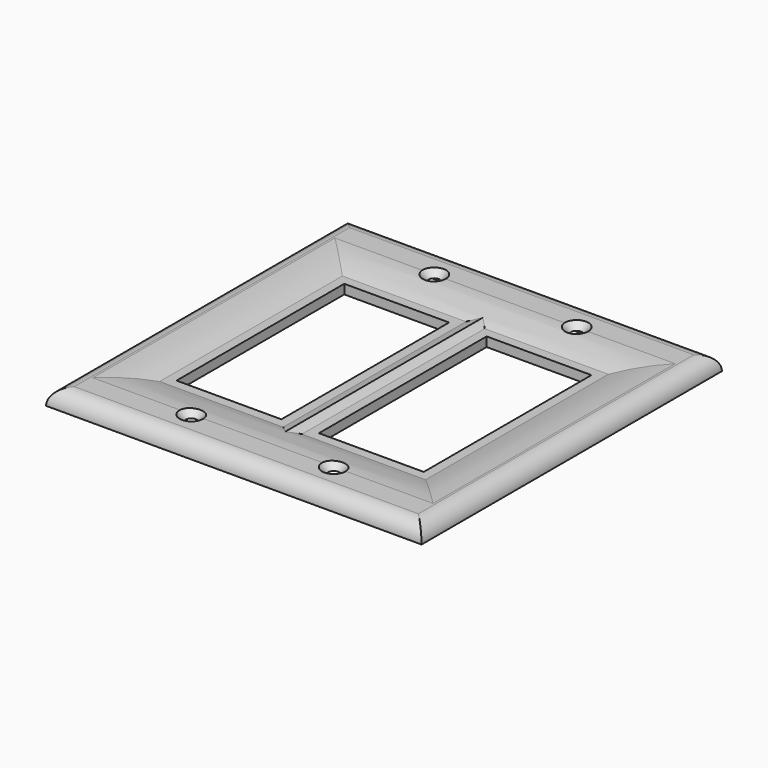
from build123d import *

# Parameters (mm, degrees)
F0_R          = 1.75
F0_W          = 39.5000008941
F0_H          = 73.0000008941
F0_W_2        = 33.5
F0_H_2        = 67
F1_DEPTH      = 5
F2_DEPTH      = 3
F3_R          = 4.99999
F4_R          = 1.5
F5_SIZE       = 1.99999
F6_R          = 2.99999
F7_START      = 3
F7_DEPTH      = 22
F8_T1_DEPTH   = 73.0000008941
F8_T3_DEPTH   = 39.5000008941
F8_T5_DEPTH   = 39.5000008941
F8_T10_DEPTH  = 69.1703579174
F8_T15_DEPTH  = 69.1703579174
F8_T20_DEPTH  = 69.1703579174
F8_T25_DEPTH  = 69.1703579174
F8_T31_DEPTH  = 102.6703579174
F8_T35_DEPTH  = 69.1703579174
F8_T43_DEPTH  = 69.1703579174
F8_T48_DEPTH  = 102.6703579174
F8_T55_DEPTH  = 102.6703579174
F8_T59_DEPTH  = 69.1703579174
F8_T66_DEPTH  = 69.1703579174
F8_T71_DEPTH  = 102.6703579174
F8_T78_DEPTH  = 102.6703579174
F8_T82_DEPTH  = 69.1703579174
F8_T89_DEPTH  = 69.1703579174
F8_T93_DEPTH  = 102.6703579174
F8_T100_DEPTH = 69.1703579174
F8_T105_DEPTH = 102.6703579174
F8_T112_DEPTH = 102.6703579174
F8_T116_DEPTH = 69.1703579174


# Not quite as in the source:
# - a fillet or chamfer that OpenCascade refuses, or shapes differently, is made with other operations: its cross-section is extruded or revolved along the edge and cut away or added
# - a fillet or chamfer is up to 0.001 mm smaller than in the source, because OpenCascade refuses the exact size
# - a feature names something its author has since deleted; it is built from what else it names


with BuildPart() as f1:
    # F0 (on Top) → F1 (new body)
    with BuildSketch(Plane.XY):
        Polygon((-60, -60), (60, -60), (60, 60), (-6, 60), (-60, 60), align=None)
        Polygon((-54.0000014007, 54.0000014007), (-6, 54.0000014007), (54.0000014007, 54.0000014007), (54.0000014007, -54.0000014007), (-54.0000014007, -54.0000014007), align=None, mode=Mode.SUBTRACT)
        Polygon((54.0000014007, 54.0000014007), (-6, 54.0000014007), (-54.0000014007, 54.0000014007), (-54.0000014007, -54.0000014007), (54.0000014007, -54.0000014007), align=None)
        with Locations((-22.75, -48.5)):
            Circle(F0_R, mode=Mode.SUBTRACT)
        with Locations((22.75, -48.5)):
            Circle(F0_R, mode=Mode.SUBTRACT)
        Polygon((-42.500000447, 36.500000447), (-6, 36.500000447), (-2.999999553, 36.500000447), (-2.999999553, -36.500000447), (-42.500000447, -36.500000447), align=None, mode=Mode.SUBTRACT)
        with Locations((-22.75, 48.5)):
            Circle(F0_R, mode=Mode.SUBTRACT)
        with Locations((22.75, 0)):
            Rectangle(F0_W, F0_H, mode=Mode.SUBTRACT)
        with Locations((22.75, 48.5)):
            Circle(F0_R, mode=Mode.SUBTRACT)
        Polygon((-2.999999553, 36.500000447), (-6, 36.500000447), (-42.500000447, 36.500000447), (-42.500000447, -36.500000447), (-2.999999553, -36.500000447), align=None)
        with Locations((-22.75, 0)):
            Rectangle(F0_W_2, F0_H_2, mode=Mode.SUBTRACT)
        with Locations((22.75, 0)):
            Rectangle(F0_W, F0_H)
        with Locations((22.75, 0)):
            Rectangle(F0_W_2, F0_H_2, mode=Mode.SUBTRACT)
    extrude(amount=F1_DEPTH)

    # F0 (on Top) → F2 (cut)
    with BuildSketch(Plane.XY):
        Polygon((54.0000014007, 54.0000014007), (-6, 54.0000014007), (-54.0000014007, 54.0000014007), (-54.0000014007, -54.0000014007), (54.0000014007, -54.0000014007), align=None)
        with Locations((-22.75, -48.5)):
            Circle(F0_R, mode=Mode.SUBTRACT)
        with Locations((22.75, -48.5)):
            Circle(F0_R, mode=Mode.SUBTRACT)
        Polygon((-42.500000447, 36.500000447), (-6, 36.500000447), (-2.999999553, 36.500000447), (-2.999999553, -36.500000447), (-42.500000447, -36.500000447), align=None, mode=Mode.SUBTRACT)
        with Locations((-22.75, 48.5)):
            Circle(F0_R, mode=Mode.SUBTRACT)
        with Locations((22.75, 0)):
            Rectangle(F0_W, F0_H, mode=Mode.SUBTRACT)
        with Locations((22.75, 48.5)):
            Circle(F0_R, mode=Mode.SUBTRACT)
    extrude(amount=F2_DEPTH, mode=Mode.SUBTRACT)

    # F3 (radius 5 in the source; OpenCascade refuses exactly that, so slightly less here)
    f3_edges = [f1.edges().sort_by_distance(p)[0] for p in [
        (0, -60, 5),
        (60, 0, 5),
        (-60, 0, 5),
        (0, 60, 5),
    ]]
    fillet(f3_edges, radius=F3_R)

    # F4
    f4_edges = [f1.edges().sort_by_distance(p)[0] for p in [
        (0, 54.000001, 3),
        (54.000001, 0, 3),
        (0, -54.000001, 3),
        (-54.000001, 0, 3),
    ]]
    fillet(f4_edges, radius=F4_R)

    # F5 (size 2 in the source; OpenCascade refuses exactly that, so slightly less here)
    f5_edges = [f1.edges().sort_by_distance(p)[0] for p in [
        (-24.5, -48.5, 5),
        (21, -48.5, 5),
        (-24.5, 48.5, 5),
        (21, 48.5, 5),
    ]]
    chamfer(f5_edges, length=F5_SIZE)

    # F6 (radius 3 in the source; OpenCascade refuses exactly that, so slightly less here)
    f6_edges = [f1.edges().sort_by_distance(p)[0] for p in [
        (22.75, 36.5, 3),
        (42.5, 0, 3),
        (-22.75, 36.5, 3),
        (-42.5, 0, 3),
        (-22.75, -36.5, 3),
        (22.75, -36.5, 3),
        (3, 0, 3),
        (-3, 0, 3),
    ]]
    fillet(f6_edges, radius=F6_R)

    # F0 (on Top) → F7 (cut)
    with BuildSketch(Plane.XY.offset(F7_START)):
        Polygon((-2.999999553, 36.500000447), (-6, 36.500000447), (-42.500000447, 36.500000447), (-42.500000447, -36.500000447), (-2.999999553, -36.500000447), align=None)
        with Locations((-22.75, 0)):
            Rectangle(F0_W_2, F0_H_2, mode=Mode.SUBTRACT)
        with Locations((22.75, 0)):
            Rectangle(F0_W, F0_H)
        with Locations((22.75, 0)):
            Rectangle(F0_W_2, F0_H_2, mode=Mode.SUBTRACT)
    extrude(amount=F7_DEPTH, mode=Mode.SUBTRACT)

    # F8: fillet of radius 36.2132034356 on 8 edges, made by hand

    # F8_s2 → F8_t1 (cut)
    with BuildSketch(Plane.XZ.offset(-36.500000447)):
        with BuildLine():
            ThreePointArc((-8.8681432564, 5), (-2.8504025312, 4.4964997224), (2.999999553, 3))
            Line((2.999999553, 3), (2.999999553, 5))
            Line((2.999999553, 5), (-8.8681432564, 5))
        make_face()
        with BuildLine():
            ThreePointArc((-54.3681432564, 5), (-48.3504025312, 4.4964997224), (-42.500000447, 3))
            Line((-42.500000447, 3), (-42.500000447, 5))
            Line((-42.500000447, 5), (-54.3681432564, 5))
        make_face()
        with BuildLine():
            ThreePointArc((54.3681432564, 5), (48.3504025312, 4.4964997224), (42.500000447, 3))
            Line((42.500000447, 3), (42.500000447, 5))
            Line((42.500000447, 5), (54.3681432564, 5))
        make_face()
        with BuildLine():
            ThreePointArc((8.8681432564, 5), (2.8504025312, 4.4964997224), (-2.999999553, 3))
            Line((-2.999999553, 3), (-2.999999553, 5))
            Line((-2.999999553, 5), (8.8681432564, 5))
        make_face()
    extrude(amount=F8_T1_DEPTH, mode=Mode.SUBTRACT)

    # F8_s4 → F8_t3 (cut)
    with BuildSketch(Plane.YZ.offset(2.999999553)):
        with BuildLine():
            ThreePointArc((-48.3681432564, 5), (-42.3504025312, 4.4964997224), (-36.500000447, 3))
            Line((-36.500000447, 3), (-36.500000447, 5))
            Line((-36.500000447, 5), (-48.3681432564, 5))
        make_face()
        with BuildLine():
            ThreePointArc((48.3681432564, 5), (42.3504025312, 4.4964997224), (36.500000447, 3))
            Line((36.500000447, 3), (36.500000447, 5))
            Line((36.500000447, 5), (48.3681432564, 5))
        make_face()
    extrude(amount=F8_T3_DEPTH, mode=Mode.SUBTRACT)

    # F8_s6 → F8_t5 (cut)
    with BuildSketch(Plane.YZ.offset(-42.500000447)):
        with BuildLine():
            ThreePointArc((-48.3681432564, 5), (-42.3504025312, 4.4964997224), (-36.500000447, 3))
            Line((-36.500000447, 3), (-36.500000447, 5))
            Line((-36.500000447, 5), (-48.3681432564, 5))
        make_face()
        with BuildLine():
            ThreePointArc((48.3681432564, 5), (42.3504025312, 4.4964997224), (36.500000447, 3))
            Line((36.500000447, 3), (36.500000447, 5))
            Line((36.500000447, 5), (48.3681432564, 5))
        make_face()
    extrude(amount=F8_T5_DEPTH, mode=Mode.SUBTRACT)


with BuildPart() as f8_tool8:
    # F8_s9 → F8_t10 (new body)
    with BuildSketch(Plane.YZ.offset(42.500000447)):
        with BuildLine():
            ThreePointArc((-48.3681432564, 5), (-42.3504025312, 4.4964997224), (-36.500000447, 3))
            Line((-36.500000447, 3), (-36.500000447, 5))
            Line((-36.500000447, 5), (-48.3681432564, 5))
        make_face()
    extrude(amount=-F8_T10_DEPTH)

    split(bisect_by=Plane.YZ.offset(-2.999999553), keep=Keep.BOTTOM)


with BuildPart() as f1_1:
    add(f1.part)

    # F8_t7: cut F8_tool8
    add(f8_tool8.part, mode=Mode.SUBTRACT)


with BuildPart() as f8_tool13:
    # F8_s14 → F8_t15 (new body)
    with BuildSketch(Plane.YZ.offset(26.6703574704)):
        with BuildLine():
            ThreePointArc((-48.3681432564, 5), (-42.3504025312, 4.4964997224), (-36.500000447, 3))
            Line((-36.500000447, 3), (-36.500000447, 5))
            Line((-36.500000447, 5), (-48.3681432564, 5))
        make_face()
    extrude(amount=-F8_T15_DEPTH)

    split(bisect_by=Plane.YZ.offset(2.999999553), keep=Keep.TOP)


with BuildPart() as f1_2:
    add(f1_1.part)

    # F8_t12: cut F8_tool13
    add(f8_tool13.part, mode=Mode.SUBTRACT)


with BuildPart() as f8_tool18:
    # F8_s19 → F8_t20 (new body)
    with BuildSketch(Plane.YZ.offset(-42.500000447)):
        with BuildLine():
            ThreePointArc((48.3681432564, 5), (42.3504025312, 4.4964997224), (36.500000447, 3))
            Line((36.500000447, 3), (36.500000447, 5))
            Line((36.500000447, 5), (48.3681432564, 5))
        make_face()
    extrude(amount=F8_T20_DEPTH)

    split(bisect_by=Plane.YZ.offset(2.999999553), keep=Keep.TOP)


with BuildPart() as f1_3:
    add(f1_2.part)

    # F8_t17: cut F8_tool18
    add(f8_tool18.part, mode=Mode.SUBTRACT)


with BuildPart() as f8_tool23:
    # F8_s24 → F8_t25 (new body)
    with BuildSketch(Plane.YZ.offset(-26.6703574704)):
        with BuildLine():
            ThreePointArc((48.3681432564, 5), (42.3504025312, 4.4964997224), (36.500000447, 3))
            Line((36.500000447, 3), (36.500000447, 5))
            Line((36.500000447, 5), (48.3681432564, 5))
        make_face()
    extrude(amount=F8_T25_DEPTH)

    split(bisect_by=Plane.YZ.offset(-2.999999553), keep=Keep.BOTTOM)


with BuildPart() as f1_4:
    add(f1_3.part)

    # F8_t22: cut F8_tool23
    add(f8_tool23.part, mode=Mode.SUBTRACT)


with BuildPart() as f8_tool29:
    # F8_s30 → F8_t31 (new body)
    with BuildSketch(Plane.XZ.offset(66.1703574704)):
        with BuildLine():
            ThreePointArc((-8.8681432564, 5), (-2.8504025312, 4.4964997224), (2.999999553, 3))
            Line((2.999999553, 3), (2.999999553, 5))
            Line((2.999999553, 5), (-8.8681432564, 5))
        make_face()
    extrude(amount=-F8_T31_DEPTH)

    split(bisect_by=Plane.XZ.offset(36.500000447), keep=Keep.TOP)


with BuildPart() as f8_tool33:
    # F8_s34 → F8_t35 (new body)
    with BuildSketch(Plane.YZ.offset(42.500000447)):
        with BuildLine():
            ThreePointArc((-48.3681432564, 5), (-42.3504025312, 4.4964997224), (-36.500000447, 3))
            Line((-36.500000447, 3), (-36.500000447, 5))
            Line((-36.500000447, 5), (-48.3681432564, 5))
        make_face()
    extrude(amount=-F8_T35_DEPTH)

    split(bisect_by=Plane.YZ.offset(2.999999553), keep=Keep.BOTTOM)

    split(bisect_by=Plane.YZ.offset(-2.999999553), keep=Keep.TOP)


with BuildPart() as f8_tool29_1:
    add(f8_tool29.part)

    # F8_t38: intersect F8_tool33
    add(f8_tool33.part, mode=Mode.INTERSECT)


with BuildPart() as f1_5:
    add(f1_4.part)

    # F8_t27: cut F8_tool29
    add(f8_tool29_1.part, mode=Mode.SUBTRACT)


with BuildPart() as f8_tool41:
    # F8_s42 → F8_t43 (new body)
    with BuildSketch(Plane.YZ.offset(-26.6703574704)):
        with BuildLine():
            ThreePointArc((48.3681432564, 5), (42.3504025312, 4.4964997224), (36.500000447, 3))
            Line((36.500000447, 3), (36.500000447, 5))
            Line((36.500000447, 5), (48.3681432564, 5))
        make_face()
    extrude(amount=F8_T43_DEPTH)

    split(bisect_by=Plane.YZ.offset(2.999999553), keep=Keep.BOTTOM)

    split(bisect_by=Plane.YZ.offset(-2.999999553), keep=Keep.TOP)


with BuildPart() as f8_tool46:
    # F8_s47 → F8_t48 (new body)
    with BuildSketch(Plane.XZ.offset(36.500000447)):
        with BuildLine():
            ThreePointArc((-8.8681432564, 5), (-2.8504025312, 4.4964997224), (2.999999553, 3))
            Line((2.999999553, 3), (2.999999553, 5))
            Line((2.999999553, 5), (-8.8681432564, 5))
        make_face()
    extrude(amount=-F8_T48_DEPTH)

    split(bisect_by=Plane.XZ.offset(-36.500000447), keep=Keep.BOTTOM)


with BuildPart() as f8_tool41_1:
    add(f8_tool41.part)

    # F8_t50: intersect F8_tool46
    add(f8_tool46.part, mode=Mode.INTERSECT)


with BuildPart() as f1_6:
    add(f1_5.part)

    # F8_t39: cut F8_tool41
    add(f8_tool41_1.part, mode=Mode.SUBTRACT)


with BuildPart() as f8_tool53:
    # F8_s54 → F8_t55 (new body)
    with BuildSketch(Plane.XZ.offset(-36.500000447)):
        with BuildLine():
            ThreePointArc((54.3681432564, 5), (48.3504025312, 4.4964997224), (42.500000447, 3))
            Line((42.500000447, 3), (42.500000447, 5))
            Line((42.500000447, 5), (54.3681432564, 5))
        make_face()
    extrude(amount=F8_T55_DEPTH)

    split(bisect_by=Plane.XZ.offset(36.500000447), keep=Keep.TOP)


with BuildPart() as f8_tool57:
    # F8_s58 → F8_t59 (new body)
    with BuildSketch(Plane.YZ.offset(72.1703574704)):
        with BuildLine():
            ThreePointArc((-48.3681432564, 5), (-42.3504025312, 4.4964997224), (-36.500000447, 3))
            Line((-36.500000447, 3), (-36.500000447, 5))
            Line((-36.500000447, 5), (-48.3681432564, 5))
        make_face()
    extrude(amount=-F8_T59_DEPTH)

    split(bisect_by=Plane.YZ.offset(42.500000447), keep=Keep.TOP)


with BuildPart() as f8_tool53_1:
    add(f8_tool53.part)

    # F8_t61: intersect F8_tool57
    add(f8_tool57.part, mode=Mode.INTERSECT)


with BuildPart() as f1_7:
    add(f1_6.part)

    # F8_t51: cut F8_tool53
    add(f8_tool53_1.part, mode=Mode.SUBTRACT)


with BuildPart() as f8_tool64:
    # F8_s65 → F8_t66 (new body)
    with BuildSketch(Plane.YZ.offset(26.6703574704)):
        with BuildLine():
            ThreePointArc((-48.3681432564, 5), (-42.3504025312, 4.4964997224), (-36.500000447, 3))
            Line((-36.500000447, 3), (-36.500000447, 5))
            Line((-36.500000447, 5), (-48.3681432564, 5))
        make_face()
    extrude(amount=-F8_T66_DEPTH)

    split(bisect_by=Plane.YZ.offset(2.999999553), keep=Keep.BOTTOM)

    split(bisect_by=Plane.YZ.offset(-2.999999553), keep=Keep.TOP)


with BuildPart() as f8_tool69:
    # F8_s70 → F8_t71 (new body)
    with BuildSketch(Plane.XZ.offset(-36.500000447)):
        with BuildLine():
            ThreePointArc((8.8681432564, 5), (2.8504025312, 4.4964997224), (-2.999999553, 3))
            Line((-2.999999553, 3), (-2.999999553, 5))
            Line((-2.999999553, 5), (8.8681432564, 5))
        make_face()
    extrude(amount=F8_T71_DEPTH)

    split(bisect_by=Plane.XZ.offset(36.500000447), keep=Keep.TOP)


with BuildPart() as f8_tool64_1:
    add(f8_tool64.part)

    # F8_t73: intersect F8_tool69
    add(f8_tool69.part, mode=Mode.INTERSECT)


with BuildPart() as f1_8:
    add(f1_7.part)

    # F8_t62: cut F8_tool64
    add(f8_tool64_1.part, mode=Mode.SUBTRACT)


with BuildPart() as f8_tool76:
    # F8_s77 → F8_t78 (new body)
    with BuildSketch(Plane.XZ.offset(66.1703574704)):
        with BuildLine():
            ThreePointArc((-54.3681432564, 5), (-48.3504025312, 4.4964997224), (-42.500000447, 3))
            Line((-42.500000447, 3), (-42.500000447, 5))
            Line((-42.500000447, 5), (-54.3681432564, 5))
        make_face()
    extrude(amount=-F8_T78_DEPTH)

    split(bisect_by=Plane.XZ.offset(36.500000447), keep=Keep.TOP)


with BuildPart() as f8_tool80:
    # F8_s81 → F8_t82 (new body)
    with BuildSketch(Plane.YZ.offset(-2.999999553)):
        with BuildLine():
            ThreePointArc((-48.3681432564, 5), (-42.3504025312, 4.4964997224), (-36.500000447, 3))
            Line((-36.500000447, 3), (-36.500000447, 5))
            Line((-36.500000447, 5), (-48.3681432564, 5))
        make_face()
    extrude(amount=-F8_T82_DEPTH)

    split(bisect_by=Plane.YZ.offset(-42.500000447), keep=Keep.BOTTOM)


with BuildPart() as f8_tool76_1:
    add(f8_tool76.part)

    # F8_t84: intersect F8_tool80
    add(f8_tool80.part, mode=Mode.INTERSECT)


with BuildPart() as f1_9:
    add(f1_8.part)

    # F8_t74: cut F8_tool76
    add(f8_tool76_1.part, mode=Mode.SUBTRACT)


with BuildPart() as f8_tool87:
    # F8_s88 → F8_t89 (new body)
    with BuildSketch(Plane.YZ.offset(-72.1703574704)):
        with BuildLine():
            ThreePointArc((48.3681432564, 5), (42.3504025312, 4.4964997224), (36.500000447, 3))
            Line((36.500000447, 3), (36.500000447, 5))
            Line((36.500000447, 5), (48.3681432564, 5))
        make_face()
    extrude(amount=F8_T89_DEPTH)

    split(bisect_by=Plane.YZ.offset(-42.500000447), keep=Keep.BOTTOM)


with BuildPart() as f8_tool91:
    # F8_s92 → F8_t93 (new body)
    with BuildSketch(Plane.XZ.offset(36.500000447)):
        with BuildLine():
            ThreePointArc((-54.3681432564, 5), (-48.3504025312, 4.4964997224), (-42.500000447, 3))
            Line((-42.500000447, 3), (-42.500000447, 5))
            Line((-42.500000447, 5), (-54.3681432564, 5))
        make_face()
    extrude(amount=-F8_T93_DEPTH)

    split(bisect_by=Plane.XZ.offset(-36.500000447), keep=Keep.BOTTOM)


with BuildPart() as f8_tool87_1:
    add(f8_tool87.part)

    # F8_t95: intersect F8_tool91
    add(f8_tool91.part, mode=Mode.INTERSECT)


with BuildPart() as f1_10:
    add(f1_9.part)

    # F8_t85: cut F8_tool87
    add(f8_tool87_1.part, mode=Mode.SUBTRACT)


with BuildPart() as f8_tool98:
    # F8_s99 → F8_t100 (new body)
    with BuildSketch(Plane.YZ.offset(-42.500000447)):
        with BuildLine():
            ThreePointArc((48.3681432564, 5), (42.3504025312, 4.4964997224), (36.500000447, 3))
            Line((36.500000447, 3), (36.500000447, 5))
            Line((36.500000447, 5), (48.3681432564, 5))
        make_face()
    extrude(amount=F8_T100_DEPTH)

    split(bisect_by=Plane.YZ.offset(2.999999553), keep=Keep.BOTTOM)

    split(bisect_by=Plane.YZ.offset(-2.999999553), keep=Keep.TOP)


with BuildPart() as f8_tool103:
    # F8_s104 → F8_t105 (new body)
    with BuildSketch(Plane.XZ.offset(-66.1703574704)):
        with BuildLine():
            ThreePointArc((8.8681432564, 5), (2.8504025312, 4.4964997224), (-2.999999553, 3))
            Line((-2.999999553, 3), (-2.999999553, 5))
            Line((-2.999999553, 5), (8.8681432564, 5))
        make_face()
    extrude(amount=F8_T105_DEPTH)

    split(bisect_by=Plane.XZ.offset(-36.500000447), keep=Keep.BOTTOM)


with BuildPart() as f8_tool98_1:
    add(f8_tool98.part)

    # F8_t107: intersect F8_tool103
    add(f8_tool103.part, mode=Mode.INTERSECT)


with BuildPart() as f1_11:
    add(f1_10.part)

    # F8_t96: cut F8_tool98
    add(f8_tool98_1.part, mode=Mode.SUBTRACT)


with BuildPart() as f8_tool110:
    # F8_s111 → F8_t112 (new body)
    with BuildSketch(Plane.XZ.offset(-66.1703574704)):
        with BuildLine():
            ThreePointArc((54.3681432564, 5), (48.3504025312, 4.4964997224), (42.500000447, 3))
            Line((42.500000447, 3), (42.500000447, 5))
            Line((42.500000447, 5), (54.3681432564, 5))
        make_face()
    extrude(amount=F8_T112_DEPTH)

    split(bisect_by=Plane.XZ.offset(-36.500000447), keep=Keep.BOTTOM)


with BuildPart() as f8_tool114:
    # F8_s115 → F8_t116 (new body)
    with BuildSketch(Plane.YZ.offset(2.999999553)):
        with BuildLine():
            ThreePointArc((48.3681432564, 5), (42.3504025312, 4.4964997224), (36.500000447, 3))
            Line((36.500000447, 3), (36.500000447, 5))
            Line((36.500000447, 5), (48.3681432564, 5))
        make_face()
    extrude(amount=F8_T116_DEPTH)

    split(bisect_by=Plane.YZ.offset(42.500000447), keep=Keep.TOP)


with BuildPart() as f8_tool110_1:
    add(f8_tool110.part)

    # F8_t118: intersect F8_tool114
    add(f8_tool114.part, mode=Mode.INTERSECT)


with BuildPart() as f1_12:
    add(f1_11.part)

    # F8_t108: cut F8_tool110
    add(f8_tool110_1.part, mode=Mode.SUBTRACT)


solid = f1_12.part
